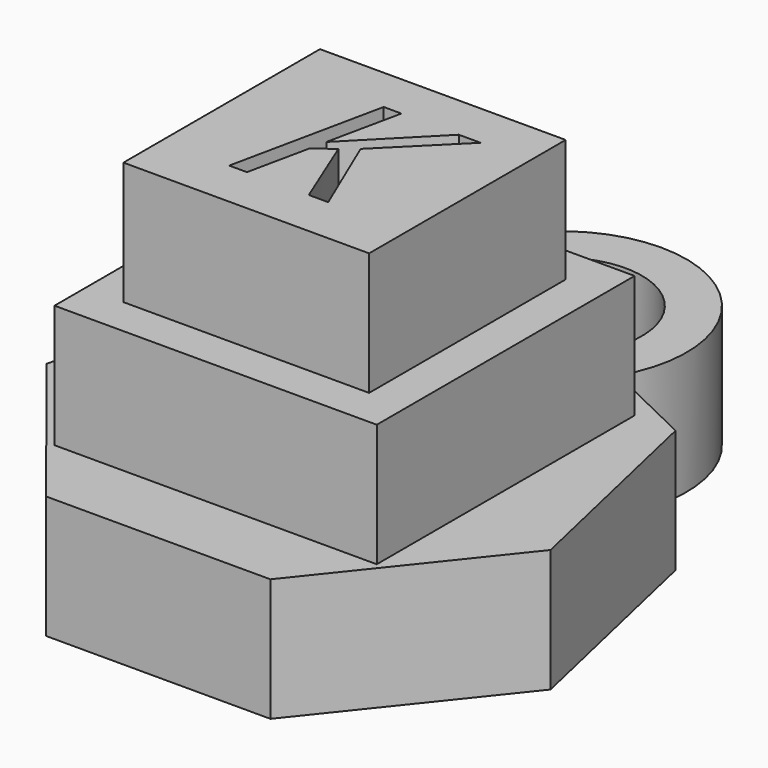
from build123d import *

# Parameters (mm, degrees)
F1_DEPTH     = 6.35
F2_W         = 16.6586078703
F2_H         = 16.6586078703
F3_DEPTH     = 6.35
F4_W         = 12.7
F4_H         = 12.7
F5_DEPTH     = 6.35
F6_TEXT_SIZE = 11.0598342467
F8_DEPTH     = 12.7
F9_R         = 6.5301019741
F9_R_2       = 4.2235943918
F10_DEPTH    = 6.35


# Not quite as in the source:
# - a feature of the source that left no trace in its solid (it failed there, or was rolled back) is left out
# - Text() gives the source's letters only with a copy of the font that has no kerning and outlines rounded to 1/6400 em; it was checked with that copy


with BuildPart() as f1:
    # F0 (on Top) → F1 (new body)
    with BuildSketch(Plane.XY):
        Polygon((5.7973842495, -12.0383924383), (13.0266041636, -2.9732373938), (10.4465254482, 8.3308260512), (0, 13.3616075617), (-10.4465254482, 8.3308260512), (-13.0266041636, -2.9732373938), (-5.7973842495, -12.0383924383), align=None)
    extrude(amount=F1_DEPTH)

    # F2 (on face) → F3 (join)
    with BuildSketch(Plane.XY.offset(6.35)):
        Rectangle(F2_W, F2_H)
    extrude(amount=F3_DEPTH)

    # F9 (on Top) → F10 (join)
    with BuildSketch(Plane.XY):
        with Locations((0, 13.9353908598)):
            Circle(F9_R)
        with Locations((0, 13.9353908598)):
            Circle(F9_R_2, mode=Mode.SUBTRACT)
    extrude(amount=F10_DEPTH)


with BuildPart() as f5:
    # F4 (on face) → F5 (new body)
    with BuildSketch(Plane.XY.offset(12.7)):
        Rectangle(F4_W, F4_H)
    extrude(amount=F5_DEPTH)

    # F6 (on face) → F8 (cut)
    with BuildSketch(Plane.XY.offset(19.05)):
        with Locations((-3.3179502934, -3.8867418189)):
            Text('K', F6_TEXT_SIZE, font='Open Sans', font_style=FontStyle.ITALIC, text_align=(TextAlign.LEFT, TextAlign.BOTTOM))
    extrude(amount=-F8_DEPTH, mode=Mode.SUBTRACT)


solid = Compound([f1.part, f5.part])
